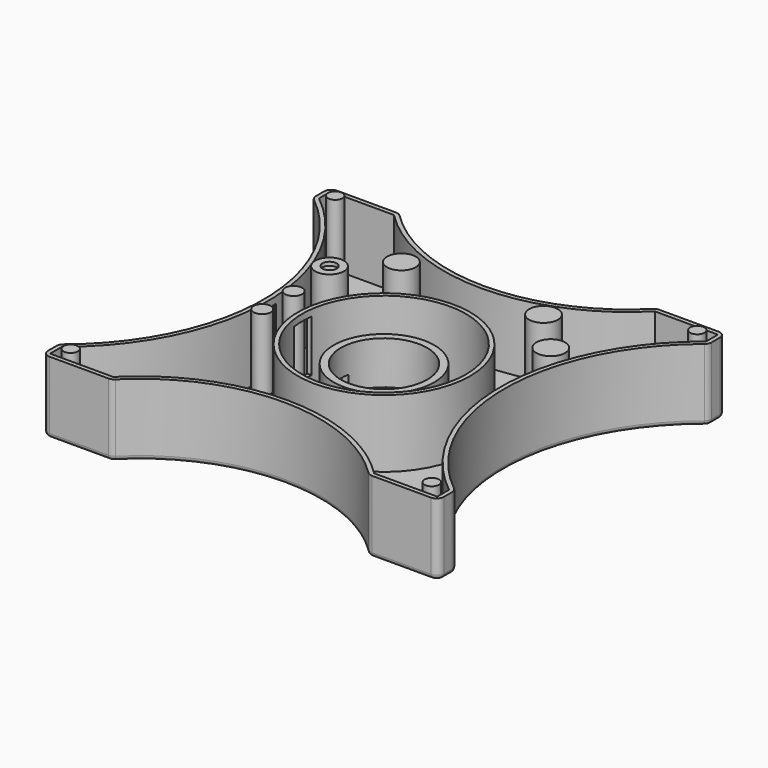
from build123d import *

# Parameters (mm, degrees)
F1_DEPTH  = 50
F2_T      = -3
F3_R      = 5
F4_R      = 60
F5_DEPTH  = 50
F6_T      = -3
F7_W      = 15.1785463095
F7_H      = 35.9015911818
F8_DEPTH  = 106.20223
F9_R      = 10
F9_R_2    = 5.9673908864
F10_DEPTH = 50
F11_R     = 5
F12_DEPTH = 2.5
F13_R     = 35
F14_DEPTH = 35
F15_T     = -5
F16_R     = 48
F17_DEPTH = 5
F18_R     = 5
F19_DEPTH = 50
F20_R     = 2.99999
F21_W     = 12.0203521578
F21_H     = 38.7059021741
F22_DEPTH = 396


# Not quite as in the source:
# - a fillet or chamfer is up to 0.001 mm smaller than in the source, because OpenCascade refuses the exact size
# - an extrude ends at something that could not be found from the text; its depth is read off the source's solid


with BuildPart() as f1:
    # F0 (on Top) → F1 (new body)
    with BuildSketch(Plane.XY):
        with BuildLine():
            Line((89.4995581526, -125), (137.647071664, -125))
            Line((137.647071664, -125), (137.647071664, -110.3164004138))
            ThreePointArc((137.647071664, -110.3164004138), (83.8462120295, 0), (137.647071664, 110.3164004138))
            Line((137.647071664, 110.3164004138), (137.647071664, 125))
            Line((137.647071664, 125), (89.4995581526, 125))
            ThreePointArc((89.4995581526, 125), (0, 87.2629880905), (-89.4995581526, 125))
            Line((-89.4995581526, 125), (-137.647071664, 125))
            Line((-137.647071664, 125), (-137.647071664, 110.3164004138))
            ThreePointArc((-137.647071664, 110.3164004138), (-83.8462120295, 0), (-137.647071664, -110.3164004138))
            Line((-137.647071664, -110.3164004138), (-137.647071664, -125))
            Line((-137.647071664, -125), (-89.4995581526, -125))
            ThreePointArc((-89.4995581526, -125), (0, -87.2629880905), (89.4995581526, -125))
        make_face()
    extrude(amount=F1_DEPTH)

    # F2
    f2_openings = [f1.faces().sort_by_distance(p)[0] for p in [
        (0, 0, 50),
    ]]
    offset(amount=F2_T, openings=f2_openings)

    # F3
    f3_edges = [f1.edges().sort_by_distance(p)[0] for p in [
        (-137.647072, -125, 25),
        (-89.499558, -125, 25),
        (89.499558, -125, 25),
        (137.647072, -125, 25),
        (137.647072, -110.3164, 25),
        (137.647072, 110.3164, 25),
        (137.647072, 125, 25),
        (89.499558, 125, 25),
        (-89.499558, 125, 25),
        (-137.647072, 125, 25),
        (-137.647072, 110.3164, 25),
        (-137.647072, -110.3164, 25),
    ]]
    fillet(f3_edges, radius=F3_R)

    # F4 (on Top) → F5 (join)
    with BuildSketch(Plane.XY):
        Circle(F4_R)
    extrude(amount=F5_DEPTH)

    # F6: a shell. OpenCascade refuses it in one call, so the cavity is built on its own and cut out:
    # the body offset inwards by the wall thickness, plus a prism from it out through each open face.
    f6_core = offset(f1.part, amount=F6_T, kind=Kind.INTERSECTION, mode=Mode.PRIVATE)
    f6_exits = [f6_core.faces().sort_by_distance(p)[0] for p in [
        (0, 0, 47),
    ]]
    add(f6_core, mode=Mode.SUBTRACT)
    extrude(f6_exits, amount=-F6_T, mode=Mode.SUBTRACT)

    # F7 (on Right) → F8 (cut)
    with BuildSketch(Plane.YZ):
        with Locations((0, 27.4735186249)):
            Rectangle(F7_W, F7_H)
    extrude(amount=-F8_DEPTH, mode=Mode.SUBTRACT)

    # F9 (on face) → F10 (join)
    with BuildSketch(Plane.XY.offset(3)):
        with Locations((-49.4316754806, 76.9219902265)):
            Circle(F9_R)
        with Locations((-76.9182676464, 48.8106995034)):
            Circle(F9_R)
        with Locations((-73.7947862563, 13.6588238292)):
            Circle(F9_R_2)
        with Locations((-73.7947862563, -13.6588238292)):
            Circle(F9_R_2)
        with Locations((49.4316754806, 76.9219902265)):
            Circle(F9_R)
        with Locations((76.9182676464, 48.8106995034)):
            Circle(F9_R)
    extrude(amount=F10_DEPTH)

    # F11 (on face) → F12 (cut)
    with BuildSketch(Plane.XY.offset(53)):
        with Locations((-76.9182676464, 48.8106995034)):
            Circle(F11_R)
    extrude(amount=-F12_DEPTH, mode=Mode.SUBTRACT)

    # F18 (on face) → F19 (join)
    with BuildSketch(Plane.XY.offset(3)):
        with Locations((-126.1960268021, 115.3223440051)):
            Circle(F18_R)
        with Locations((126.1960342526, 114.7097125649)):
            Circle(F18_R)
        with Locations((-125.8897334337, -115.0275468826)):
            Circle(F18_R)
        with Locations((125.2771168947, -115.0275468826)):
            Circle(F18_R)
    extrude(amount=F19_DEPTH)

    # F20 (radius 3 in the source; OpenCascade refuses exactly that, so slightly less here)
    f20_edges = [f1.edges().sort_by_distance(p)[0] for p in [
        (112.115296, -125, 0),
        (136.182606, -123.535534, 0),
        (137.647072, -116.364255, 0),
        (137.159498, -110.574906, 0),
        (83.846212, 0, 0),
        (137.159498, 110.574906, 0),
        (137.647072, 116.364255, 0),
        (136.182606, 123.535534, 0),
        (112.115296, 125, 0),
        (89.678642, 124.622926, 0),
        (0, 87.262988, 0),
        (-89.678642, 124.622926, 0),
        (-112.115296, 125, 0),
        (-136.182606, 123.535534, 0),
        (-137.647072, 116.364255, 0),
        (-137.159498, 110.574906, 0),
        (-83.846212, 0, 0),
        (-137.159498, -110.574906, 0),
        (-137.647072, -116.364255, 0),
        (-136.182606, -123.535534, 0),
        (-112.115296, -125, 0),
        (-89.678642, -124.622926, 0),
        (0, -87.262988, 0),
        (89.678642, -124.622926, 0),
        (-84.052067, 7.589273, 27.473519),
        (-84.052067, -7.589273, 27.473519),
        (-83.846212, 0, 45.424314),
        (-83.846212, 0, 9.522723),
    ]]
    fillet(f20_edges, radius=F20_R)


with BuildPart() as f14:
    # F13 (on face) → F14 (new body)
    with BuildSketch(Plane.XY.offset(3)):
        Circle(F13_R)
    extrude(amount=F14_DEPTH)

    # F15
    f15_openings = [f14.faces().sort_by_distance(p)[0] for p in [
        (0, 0, 38),
    ]]
    offset(amount=F15_T, openings=f15_openings)

    # F16 (on face) → F17 (join)
    with BuildSketch(Plane.XY.offset(3)):
        Circle(F16_R)
    extrude(amount=F17_DEPTH)

    # F21 (on Right) → F22 (cut, through all)
    with BuildSketch(Plane.YZ):
        Rectangle(F21_W, F21_H)
    extrude(amount=-F22_DEPTH, mode=Mode.SUBTRACT)


solid = Compound([f1.part, f14.part])
